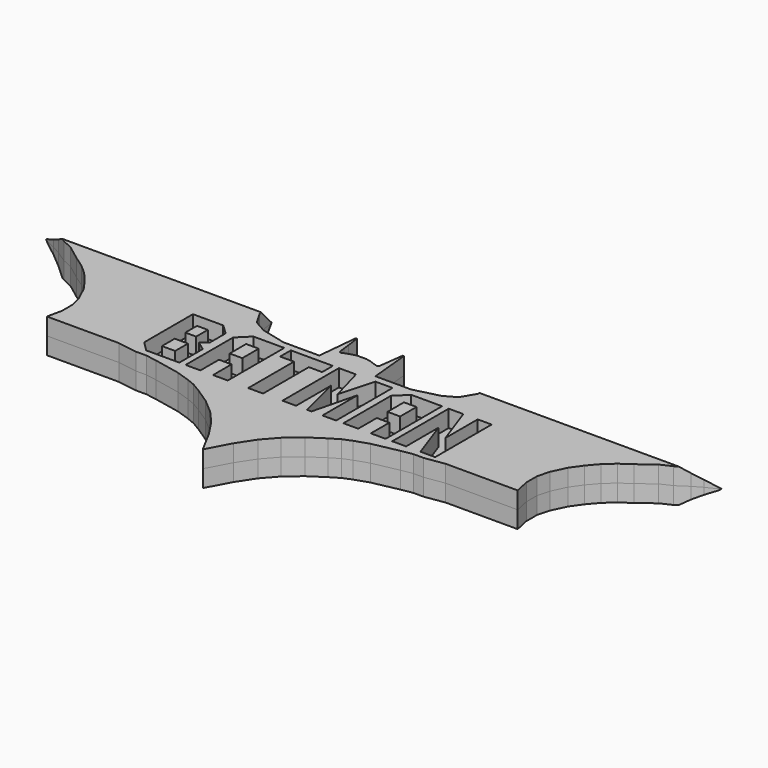
from build123d import *

# Parameters (mm, degrees)
F1_DEPTH      = 2
F2_W          = 1.5500899148
F2_H          = 1.876123564
F2_W_2        = 1.2698153506
F2_H_2        = 1.7102467797
F2_W_3        = 1.4757313342
F2_H_3        = 2.4080732306
F2_W_4        = 1.4757313005
F3_DEPTH      = 3.5
F4_DEPTH      = 2
F5_T1_DEPTH   = 39.984208449
F5_T3_DEPTH   = 39.984208449
F5_2_T1_DEPTH = 39.984208449
F5_2_T3_DEPTH = 39.984208449


# Not quite as in the source:
# - a fillet or chamfer that OpenCascade refuses, or shapes differently, is made with other operations: its cross-section is extruded or revolved along the edge and cut away or added


with BuildPart() as f1:
    # F0 (on Top) → F1 (new body)
    with BuildSketch(Plane.XY):
        Polygon((0, 1.0266449535), (0, 24.3500620127), (-0.544148148, 24.3500620127), (-1.0979532963, 24.2267251015), (-1.4955324586, 24.0809451789), (-1.8798589008, 23.9484198391), (-2.0664292388, 23.8823629916), (-2.1881915163, 23.8823629916), (-2.2490727715, 23.9484198391), (-2.3099537939, 24.0809451789), (-2.3447431158, 24.3500620127), (-2.3924632423, 24.7192065845), (-2.4914027403, 25.4845645437), (-2.6816999265, 26.9566304925), (-2.7555432171, 26.9566304925), (-2.8086215714, 26.9497689375), (-2.8312180657, 26.8769655377), (-3.287199419, 22.2009196877), (-6.5677068196, 22.2009196877), (-7.4946065433, 22.2009196877), (-8.7081333622, 22.5128047168), (-10.4070715606, 22.9288712144), (-11.8286330253, 23.7263310701), (-12.7647817135, 25.3212526441), (-13.2530452684, 28.0673876405), (-40.3788387775, 28.0673876405), (-39.3400602043, 27.4067055434), (-38.093522191, 26.7834383994), (-37.0547436178, 26.2017212808), (-35.7251018286, 25.3212526441), (-34.4370156527, 24.7192065845), (-32.6503142715, 23.376237601), (-31.4037762582, 22.5128047168), (-30.281893909, 21.5064324439), (-29.284665361, 20.3430000693), (-28.3705387264, 19.0549120307), (-27.5810658932, 17.3928625882), (-27.2071044892, 15.9801207483), (-27.2071044892, 14.4011750817), (-27.5810658932, 12.6721505076), (-26.3990871608, 12.6721505076), (-23.7930994481, 12.6721505076), (-22.6050745696, 12.6721505076), (-21.1104638875, 12.6721505076), (-19.1508084536, 12.6721505076), (-16.8494340032, 12.3221287504), (-15.6418774277, 12.3221287504), (-14.3144382164, 12.0935244486), (-11.2784868106, 11.4729851484), (-9.6770906821, 10.9391864389), (-8.6619686335, 10.5253299698), (-7.5719556771, 9.8713217303), (-5.8279349469, 8.7190223858), (-4.1462001391, 7.2864340618), (-2.7447550092, 5.6981290691), (-1.4367403928, 3.7049627863), align=None)
        Polygon((0.544148148, 24.3500620127), (0, 24.3500620127), (0, 1.0266449535), (1.4367403928, 3.7049627863), (2.7447550092, 5.6981290691), (4.1462001391, 7.2864340618), (5.8279349469, 8.7190223858), (7.5719556771, 9.8713217303), (8.6619686335, 10.5253299698), (9.6770906821, 10.9391864389), (11.2784868106, 11.4729851484), (14.3144382164, 12.0935244486), (15.6418774277, 12.3221287504), (16.8494340032, 12.3221287504), (19.1508084536, 12.6721505076), (21.1104638875, 12.6721505076), (22.6050745696, 12.6721505076), (23.7930994481, 12.6721505076), (26.3990871608, 12.6721505076), (27.5810658932, 12.6721505076), (27.2071044892, 14.4011750817), (27.2071044892, 15.9801207483), (27.5810658932, 17.3928625882), (28.3705387264, 19.0549120307), (29.284665361, 20.3430000693), (30.281893909, 21.5064324439), (31.4037762582, 22.5128047168), (32.6503142715, 23.376237601), (34.4370156527, 24.7192065845), (35.7251018286, 25.3212526441), (37.0547436178, 26.2017212808), (38.093522191, 26.7834383994), (39.3400602043, 27.4067055434), (40.3788387775, 28.0673876405), (13.2530452684, 28.0673876405), (12.7647817135, 25.3212526441), (11.8286330253, 23.7263310701), (10.4070715606, 22.9288712144), (8.7081333622, 22.5128047168), (7.4946065433, 22.2009196877), (6.5677068196, 22.2009196877), (3.287199419, 22.2009196877), (2.8312180657, 26.8769655377), (2.8086215714, 26.9497689375), (2.7555432171, 26.9566304925), (2.6816999265, 26.9566304925), (2.4914027403, 25.4845645437), (2.3924632423, 24.7192065845), (2.3447431158, 24.3500620127), (2.3099537939, 24.0809451789), (2.2490727715, 23.9484198391), (2.1881915163, 23.8823629916), (2.0664292388, 23.8823629916), (1.8798589008, 23.9484198391), (1.4955324586, 24.0809451789), (1.0979532963, 24.2267251015), align=None)
    extrude(amount=F1_DEPTH)

    # F2 (on face) → F3 (cut)
    with BuildSketch(Plane.XY.offset(2)):
        Polygon((-12.4121709659, 13.1039507687), (-12.4121709659, 16.5473238707), (-13.5275493035, 17.3538282159), (-12.7153250727, 18.005895548), (-12.7153250727, 20.2824113081), (-13.8879023002, 21.3749100694), (-17.4342334108, 21.3749100694), (-17.4342334108, 14.2479285344), (-16.2902556114, 13.1039507687), align=None)
        with Locations((-14.9260621312, 15.6092620887)):
            Rectangle(F2_W, F2_H, mode=Mode.SUBTRACT)
        with Locations((-15.0661994133, 18.946817256)):
            Rectangle(F2_W_2, F2_H_2, mode=Mode.SUBTRACT)
        Polygon((-11.6800252013, 13.1039507687), (-9.9411789934, 13.1039507687), (-9.9411789934, 15.8208979917), (-8.4654476592, 15.8208979917), (-8.4654476592, 13.1039507687), (-6.732321337, 13.1039507687), (-6.732321337, 21.3749100694), (-10.3472910751, 21.3749100694), (-11.6800252013, 20.0650555195), align=None)
        with Locations((-9.2033133263, 18.5979040305)):
            Rectangle(F2_W_3, F2_H_3, mode=Mode.SUBTRACT)
        Polygon((-2.5968416698, 19.8019406458), (-1.0353120174, 19.8019406458), (-1.0353120174, 21.3749100694), (-5.9601363392, 21.3749100694), (-5.9601363392, 19.8019406458), (-4.3414077632, 19.8019406458), (-4.3414077632, 13.1039507687), (-2.5968416698, 13.1039507687), align=None)
        Polygon((5.9601120808, 21.3749100694), (3.9581509656, 21.3749100694), (2.8141731999, 17.2565900928), (1.6701954343, 21.3749100694), (-0.3317656809, 21.3749100694), (-0.3317656809, 13.1039507687), (1.2698032045, 13.1039507687), (1.2698032045, 18.2518507648), (2.5567782119, 13.1039507687), (3.071568188, 13.1039507687), (4.3585431954, 18.2518507648), (4.3585431954, 13.1039507687), (5.9601120808, 13.1039507687), align=None)
        Polygon((6.812375511, 13.1039507687), (8.5512217526, 13.1039507687), (8.5512217526, 15.8208979917), (10.0269530531, 15.8208979917), (10.0269530531, 13.1039507687), (11.760079409, 13.1039507687), (11.760079409, 21.3749100694), (8.1451096372, 21.3749100694), (6.812375511, 20.0650555195), align=None)
        with Locations((9.2890874028, 18.5979040305)):
            Rectangle(F2_W_4, F2_H_3, mode=Mode.SUBTRACT)
        Polygon((15.92987839, 21.3749100694), (15.92987839, 16.6274023032), (14.2482310384, 21.3749100694), (12.5322644068, 21.3749100694), (12.5322644068, 13.1039507687), (14.1567128347, 13.1039507687), (14.1567128347, 17.851458535), (15.8497999238, 13.1039507687), (17.5657665892, 13.1039507687), (17.5657665892, 21.3749100694), align=None)
    extrude(amount=-F3_DEPTH, mode=Mode.SUBTRACT)

    # F5#2: chamfer of 2.5 on 2 edges, made by hand

    # F5_2_s2 → F5_2_t1 (cut)
    with BuildSketch(Plane.YZ.offset(6.8238377984)):
        Polygon((25.5673876405, 2), (28.0673876405, -0.5), (28.0673876405, 2), align=None)
    extrude(amount=F5_2_T1_DEPTH, mode=Mode.SUBTRACT)

    # F5_2_s4 → F5_2_t3 (cut)
    with BuildSketch(Plane.YZ.offset(-46.8080462475)):
        Polygon((25.5673876405, 2), (28.0673876405, -0.5), (28.0673876405, 2), align=None)
    extrude(amount=F5_2_T3_DEPTH, mode=Mode.SUBTRACT)


with BuildPart() as f4:
    # F0 (on Top) → F4 (new body)
    with BuildSketch(Plane.XY):
        Polygon((0, 1.0266449535), (0, 24.3500620127), (-0.544148148, 24.3500620127), (-1.0979532963, 24.2267251015), (-1.4955324586, 24.0809451789), (-1.8798589008, 23.9484198391), (-2.0664292388, 23.8823629916), (-2.1881915163, 23.8823629916), (-2.2490727715, 23.9484198391), (-2.3099537939, 24.0809451789), (-2.3447431158, 24.3500620127), (-2.3924632423, 24.7192065845), (-2.4914027403, 25.4845645437), (-2.6816999265, 26.9566304925), (-2.7555432171, 26.9566304925), (-2.8086215714, 26.9497689375), (-2.8312180657, 26.8769655377), (-3.287199419, 22.2009196877), (-6.5677068196, 22.2009196877), (-7.4946065433, 22.2009196877), (-8.7081333622, 22.5128047168), (-10.4070715606, 22.9288712144), (-11.8286330253, 23.7263310701), (-12.7647817135, 25.3212526441), (-13.2530452684, 28.0673876405), (-40.3788387775, 28.0673876405), (-39.3400602043, 27.4067055434), (-38.093522191, 26.7834383994), (-37.0547436178, 26.2017212808), (-35.7251018286, 25.3212526441), (-34.4370156527, 24.7192065845), (-32.6503142715, 23.376237601), (-31.4037762582, 22.5128047168), (-30.281893909, 21.5064324439), (-29.284665361, 20.3430000693), (-28.3705387264, 19.0549120307), (-27.5810658932, 17.3928625882), (-27.2071044892, 15.9801207483), (-27.2071044892, 14.4011750817), (-27.5810658932, 12.6721505076), (-26.3990871608, 12.6721505076), (-23.7930994481, 12.6721505076), (-22.6050745696, 12.6721505076), (-21.1104638875, 12.6721505076), (-19.1508084536, 12.6721505076), (-16.8494340032, 12.3221287504), (-15.6418774277, 12.3221287504), (-14.3144382164, 12.0935244486), (-11.2784868106, 11.4729851484), (-9.6770906821, 10.9391864389), (-8.6619686335, 10.5253299698), (-7.5719556771, 9.8713217303), (-5.8279349469, 8.7190223858), (-4.1462001391, 7.2864340618), (-2.7447550092, 5.6981290691), (-1.4367403928, 3.7049627863), align=None)
        Polygon((0.544148148, 24.3500620127), (0, 24.3500620127), (0, 1.0266449535), (1.4367403928, 3.7049627863), (2.7447550092, 5.6981290691), (4.1462001391, 7.2864340618), (5.8279349469, 8.7190223858), (7.5719556771, 9.8713217303), (8.6619686335, 10.5253299698), (9.6770906821, 10.9391864389), (11.2784868106, 11.4729851484), (14.3144382164, 12.0935244486), (15.6418774277, 12.3221287504), (16.8494340032, 12.3221287504), (19.1508084536, 12.6721505076), (21.1104638875, 12.6721505076), (22.6050745696, 12.6721505076), (23.7930994481, 12.6721505076), (26.3990871608, 12.6721505076), (27.5810658932, 12.6721505076), (27.2071044892, 14.4011750817), (27.2071044892, 15.9801207483), (27.5810658932, 17.3928625882), (28.3705387264, 19.0549120307), (29.284665361, 20.3430000693), (30.281893909, 21.5064324439), (31.4037762582, 22.5128047168), (32.6503142715, 23.376237601), (34.4370156527, 24.7192065845), (35.7251018286, 25.3212526441), (37.0547436178, 26.2017212808), (38.093522191, 26.7834383994), (39.3400602043, 27.4067055434), (40.3788387775, 28.0673876405), (13.2530452684, 28.0673876405), (12.7647817135, 25.3212526441), (11.8286330253, 23.7263310701), (10.4070715606, 22.9288712144), (8.7081333622, 22.5128047168), (7.4946065433, 22.2009196877), (6.5677068196, 22.2009196877), (3.287199419, 22.2009196877), (2.8312180657, 26.8769655377), (2.8086215714, 26.9497689375), (2.7555432171, 26.9566304925), (2.6816999265, 26.9566304925), (2.4914027403, 25.4845645437), (2.3924632423, 24.7192065845), (2.3447431158, 24.3500620127), (2.3099537939, 24.0809451789), (2.2490727715, 23.9484198391), (2.1881915163, 23.8823629916), (2.0664292388, 23.8823629916), (1.8798589008, 23.9484198391), (1.4955324586, 24.0809451789), (1.0979532963, 24.2267251015), align=None)
    extrude(amount=-F4_DEPTH)

    # F5: chamfer of 2.5 on 2 edges, made by hand

    # F5_s2 → F5_t1 (cut)
    with BuildSketch(Plane.YZ.offset(6.8238377984)):
        Polygon((28.0673876405, 0.5), (25.5673876405, -2), (28.0673876405, -2), align=None)
    extrude(amount=F5_T1_DEPTH, mode=Mode.SUBTRACT)

    # F5_s4 → F5_t3 (cut)
    with BuildSketch(Plane.YZ.offset(-46.8080462475)):
        Polygon((28.0673876405, 0.5), (25.5673876405, -2), (28.0673876405, -2), align=None)
    extrude(amount=F5_T3_DEPTH, mode=Mode.SUBTRACT)


solid = Compound([f1.part, f4.part])
